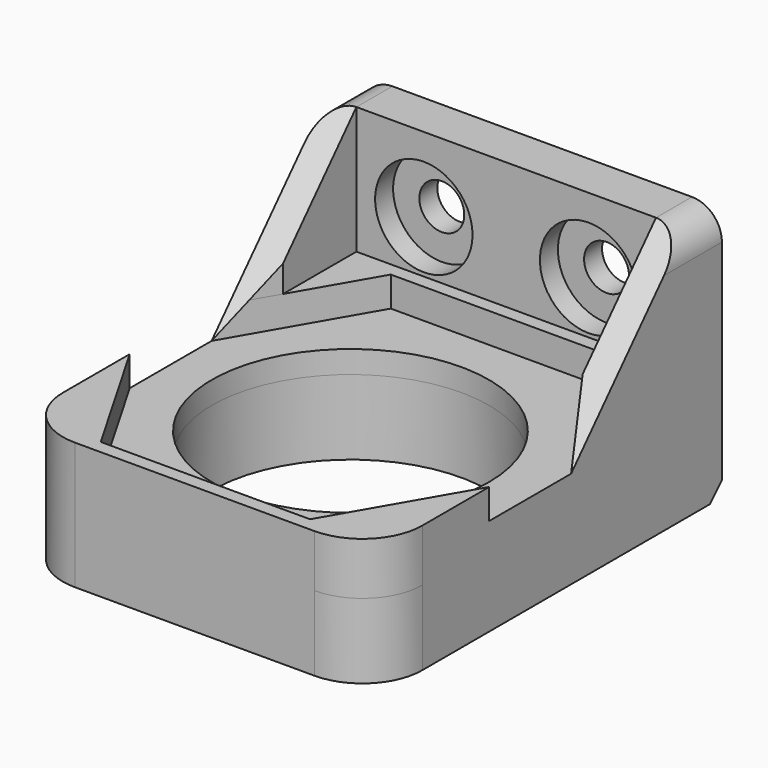
from build123d import *

# Parameters (mm, degrees)
F0_W           = 24
F0_H           = 12
F1_DEPTH       = 3
F3_D           = 3
F3_CBORE_D     = 6.5
F3_CBORE_DEPTH = 1.5
F4_DEPTH       = 26
F7_R           = 4
F8_R           = 9.25
F9_DEPTH       = 25
F10_DEPTH      = 5
F11_DEPTH      = 2
F2_W           = 2
F2_H           = 8.5
F12_REACH      = 34.7331245983
F5_W           = 2
F5_H           = 8.5
F13_REACH      = 34.7331245983
F14_SIZE       = 1
F15_R          = 2
F17_DEPTH      = 25


# Not quite as in the source:
# - a feature names something its author has since deleted; it is built from what else it names


with BuildPart() as f1:
    # F0 (on Front) → F1 (new body)
    with BuildSketch(Plane.XZ):
        with Locations((12, 6)):
            Rectangle(F0_W, F0_H)
    extrude(amount=F1_DEPTH)

    # F3 (through all)
    with Locations(Plane.XZ.offset(3)):
        with Locations((6.5, 7), (17.5, 7)):
            CounterBoreHole(F3_D / 2, F3_CBORE_D / 2, F3_CBORE_DEPTH)

    # F2 (on face) → F4 (join)
    with BuildSketch(Plane.XZ.offset(3)):
        Polygon((0, 3.5), (0, 0), (24, 0), (24, 3.5), (22, 3.5), (2, 3.5), align=None)
    extrude(amount=F4_DEPTH)

    # F7
    f7_edges = [f1.edges().sort_by_distance(p)[0] for p in [
        (24, -29, 1.75),
        (0, -29, 1.75),
    ]]
    fillet(f7_edges, radius=F7_R)

    # F8 (on face) → F9 (cut)
    with BuildSketch(Plane(origin=(0, 0, 0), x_dir=(1, 0, 0), z_dir=(0, 0, -1))):
        with Locations((12, 16)):
            Circle(F8_R)
    extrude(amount=-F9_DEPTH, mode=Mode.SUBTRACT)

    # F10 (add): a face of the model
    f10_faces = [f1.faces().sort_by_distance(p)[0] for p in [
        (0.3764306045, -12.5, 0),
    ]]
    extrude(f10_faces, amount=F10_DEPTH)

    # F6 (on face) → F11 (cut)
    with BuildSketch(Plane.XY.offset(3.5)):
        Polygon((0, -19.4153903092), (5.0140617428, -28.1), (18.9859382572, -28.1), (24, -19.4153903092), (24, -12.5846096908), (18.9859382572, -3.9), (5.0140617428, -3.9), (0, -12.5846096908), align=None)
    extrude(amount=-F11_DEPTH, mode=Mode.SUBTRACT)

    f12_end = Plane(origin=(2.5070308714, -8.2423048454, 2.5), x_dir=(0.5, 0.8660254038, 0), z_dir=(0.8660254038, -0.5, 0))
    # F2 (on face) → F12 (join, up to a plane its end follows)
    with BuildSketch(Plane.XZ.offset(3)):
        with Locations((1, 7.75)):
            Rectangle(F2_W, F2_H)
    f12_long = extrude(amount=F12_REACH, mode=Mode.PRIVATE)
    add(split(f12_long, bisect_by=f12_end, keep=Keep.BOTTOM, mode=Mode.PRIVATE))

    f13_end = Plane(origin=(21.4929691286, -8.2423048454, 2.5), x_dir=(0.5, -0.8660254038, 0), z_dir=(-0.8660254038, -0.5, 0))
    # F5 (on face) → F13 (join, up to a plane its end follows)
    with BuildSketch(Plane.XZ.offset(3)):
        with Locations((23, 7.75)):
            Rectangle(F5_W, F5_H)
    f13_long = extrude(amount=F13_REACH, mode=Mode.PRIVATE)
    add(split(f13_long, bisect_by=f13_end, keep=Keep.BOTTOM, mode=Mode.PRIVATE))

    # F14
    f14_edges = [f1.edges().sort_by_distance(p)[0] for p in [
        (12, 0, -5),
    ]]
    chamfer(f14_edges, length=F14_SIZE)

    # F15
    f15_edges = [f1.edges().sort_by_distance(p)[0] for p in [
        (24, -6.292305, 12),
        (0, -6.292305, 12),
    ]]
    fillet(f15_edges, radius=F15_R)

    # F16 (on face) → F17 (cut)
    with BuildSketch(Plane.YZ.offset(24)):
        Polygon((-12.5846096908, 12), (-12.5846096908, 1.5), (-3, 12), align=None)
    extrude(amount=-F17_DEPTH, mode=Mode.SUBTRACT)


solid = f1.part
